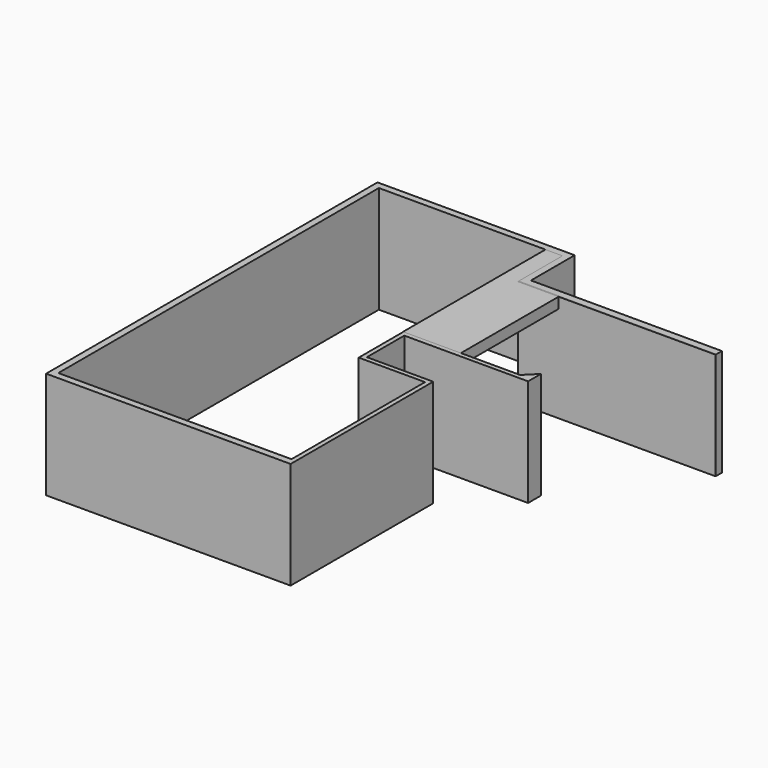
from build123d import *

# Parameters (mm, degrees)
F1_DEPTH = 2400.3
F3_W     = 381
F3_H     = 241.3
F4_DEPTH = 3987.8
F5_DEPTH = 25.4
F6_W     = 914.4
F6_H     = 241.3
F7_DEPTH = 2736.85


with BuildPart() as f1:
    # F0 (on Top) → F1 (new body)
    with BuildSketch(Plane.XY):
        Polygon((0, -8978.9), (0, 0), (4114.8, 0), (4114.8, -1225.55), (8547.1, -1225.55), (8547.1, -1073.15), (4267.2, -1073.15), (4267.2, 152.4), (-152.4, 152.4), (-152.4, -9131.3), (5327.65, -9131.3), (5327.65, -5137.15), (3841.75, -5137.15), (3841.75, -4089.4), (6616.7, -4089.4), (6616.7, -3729.1686237132), (6358.0686237132, -3987.8), (3740.15, -3987.8), (3740.15, -5238.75), (5226.05, -5238.75), (5226.05, -8978.9), align=None)
    extrude(amount=F1_DEPTH)


with BuildPart() as f4:
    # F3 (on face) → F4 (new body, through all)
    with BuildSketch(Plane.XZ):
        with Locations((3924.3, 2279.65)):
            Rectangle(F3_W, F3_H)
    extrude(amount=F4_DEPTH)

    # F6 (on face) → F7 (join, through all)
    with BuildSketch(Plane.XZ.offset(1250.95)):
        with Locations((4572, 2279.65)):
            Rectangle(F6_W, F6_H)
    extrude(amount=F7_DEPTH)


with BuildPart() as f5:
    # F5 (new): a face of the model
    f5_faces = [f1.part.faces().sort_by_distance(p)[0] for p in [
        (6330.95, -1225.55, 1200.15),
    ]]
    extrude(f5_faces, amount=F5_DEPTH)


solid = Compound([f1.part, f4.part, f5.part])
